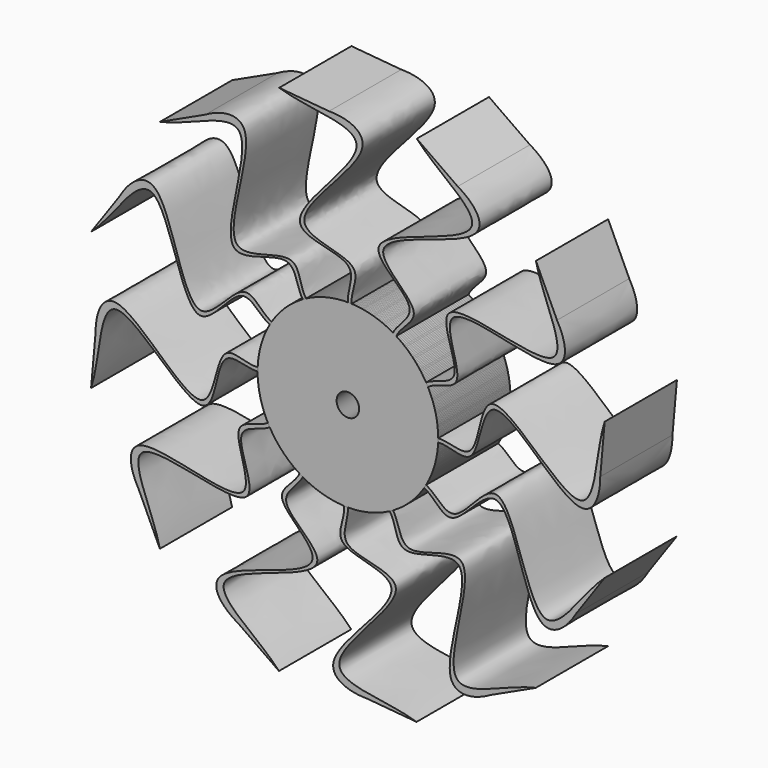
from build123d import *

# Parameters (mm, degrees)
F0_R     = 3.175
F1_DEPTH = 25.4
F2_COUNT = 12


with BuildPart() as f1:
    # F0 (on Front) → F1 (new body)
    with BuildSketch(Plane.XZ):
        with BuildLine():
            ThreePointArc((0, 25.4), (-17.9605122421, -17.9605122421), (25.4, 0))
            ThreePointArc((25.4, 0), (18.3349277735, 17.5781234363), (1.0700453904, 25.377450677))
            ThreePointArc((1.0700453904, 25.377450677), (0.5351414789, 25.3943620435), (0, 25.4))
        make_face()
        Circle(F0_R, mode=Mode.SUBTRACT)
        with BuildLine():
            ThreePointArc((0, 25.4), (0.5351414789, 25.3943620435), (1.0700453904, 25.377450677))
            Line((1.0700453904, 25.377450677), (1.0695737267, 25.4))
            Line((1.0695737267, 25.4), (0, 25.4))
        make_face()
        with BuildLine():
            add(Edge.make_bspline(
                [(0, 25.4), (-0.2214922769, 28.4921921416), (5.1320365421, 37.4454677347), (-26.6848057865, 36.6120551679), (17.6752109872, 70.931210213), (-11.3022852987, 69.5911206252), (-19.3284919004, 72.2468848729)],
                knots=[0, 0, 0, 0, 0.177403549, 0.4031983824, 0.7192037587, 1, 1, 1, 1], degree=3))
            Line((0, 25.4), (1.0695737267, 25.4))
            add(Edge.make_bspline(
                [(1.0695737267, 25.4), (0.7290682583, 28.5763884935), (6.7412665977, 37.2695244957), (-25.2200163673, 37.5073747812), (12.7550310137, 66.0371385481), (0, 71.0008963943), (-5.3024357185, 71.0008963943)],
                knots=[0, 0, 0, 0, 0.1937309868, 0.4425472111, 0.7867659207, 1, 1, 1, 1], degree=3))
            Line((-5.3024357185, 71.0008963943), (-19.3284919004, 72.2468848729))
        make_face()
    extrude(amount=-F1_DEPTH)


with BuildPart() as f2_1:
    # F2: instance of F1
    add(f1.part.rotate(Axis((0, 0, 0), (0, -1, 0)), 1 * 360 / F2_COUNT))


with BuildPart() as f2_2:
    # F2: instance of F1
    add(f1.part.rotate(Axis((0, 0, 0), (0, -1, 0)), 2 * 360 / F2_COUNT))


with BuildPart() as f2_3:
    # F2: instance of F1
    add(f1.part.rotate(Axis((0, 0, 0), (0, -1, 0)), 3 * 360 / F2_COUNT))


with BuildPart() as f2_4:
    # F2: instance of F1
    add(f1.part.rotate(Axis((0, 0, 0), (0, -1, 0)), 4 * 360 / F2_COUNT))


with BuildPart() as f2_5:
    # F2: instance of F1
    add(f1.part.rotate(Axis((0, 0, 0), (0, -1, 0)), 5 * 360 / F2_COUNT))


with BuildPart() as f2_6:
    # F2: instance of F1
    add(f1.part.rotate(Axis((0, 0, 0), (0, -1, 0)), 6 * 360 / F2_COUNT))


with BuildPart() as f2_7:
    # F2: instance of F1
    add(f1.part.rotate(Axis((0, 0, 0), (0, -1, 0)), 7 * 360 / F2_COUNT))


with BuildPart() as f2_8:
    # F2: instance of F1
    add(f1.part.rotate(Axis((0, 0, 0), (0, -1, 0)), 8 * 360 / F2_COUNT))


with BuildPart() as f2_9:
    # F2: instance of F1
    add(f1.part.rotate(Axis((0, 0, 0), (0, -1, 0)), 9 * 360 / F2_COUNT))


with BuildPart() as f2_10:
    # F2: instance of F1
    add(f1.part.rotate(Axis((0, 0, 0), (0, -1, 0)), 10 * 360 / F2_COUNT))


with BuildPart() as f2_11:
    # F2: instance of F1
    add(f1.part.rotate(Axis((0, 0, 0), (0, -1, 0)), 11 * 360 / F2_COUNT))


solid = Compound([f1.part, f2_1.part, f2_2.part, f2_3.part, f2_4.part, f2_5.part, f2_6.part, f2_7.part, f2_8.part, f2_9.part, f2_10.part, f2_11.part])
